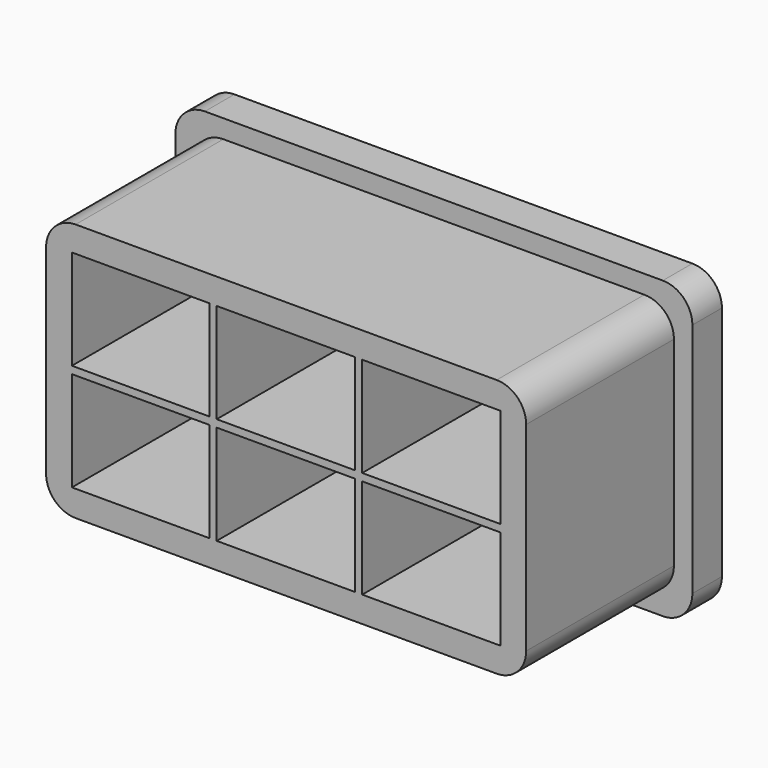
from build123d import *

# Parameters (mm, degrees)
F0_W     = 165.1
F0_H     = 88.9
F0_W_2   = 152.4
F0_H_2   = 76.2
F1_DEPTH = 76.2
F0_W_3   = 47.244
F0_H_3   = 34.29
F0_W_4   = 47.498
F2_DEPTH = 76.2
F3_R     = 10.16
F4_W     = 177.8
F4_H     = 101.6
F5_DEPTH = 12.7
F6_R     = 10.16


# Not quite as in the source:
# - a feature names something its author has since deleted; it is built from what else it names


with BuildPart() as f1:
    # F0 (on Front) → F1 (new body)
    with BuildSketch(Plane.XZ):
        Rectangle(F0_W, F0_H)
        Rectangle(F0_W_2, F0_H_2, mode=Mode.SUBTRACT)
    extrude(amount=F1_DEPTH)

    # F0 (on Front) → F2 (join)
    with BuildSketch(Plane.XZ):
        Rectangle(F0_W_2, F0_H_2)
        with Locations((-50.038, -18.415)):
            Rectangle(F0_W_3, F0_H_3, mode=Mode.SUBTRACT)
        with Locations((-0.127, -18.415)):
            Rectangle(F0_W_4, F0_H_3, mode=Mode.SUBTRACT)
        with Locations((49.911, -18.415)):
            Rectangle(F0_W_4, F0_H_3, mode=Mode.SUBTRACT)
        with Locations((-50.038, 18.415)):
            Rectangle(F0_W_3, F0_H_3, mode=Mode.SUBTRACT)
        with Locations((-0.127, 18.415)):
            Rectangle(F0_W_4, F0_H_3, mode=Mode.SUBTRACT)
        with Locations((49.911, 18.415)):
            Rectangle(F0_W_4, F0_H_3, mode=Mode.SUBTRACT)
    extrude(amount=F2_DEPTH)

    # F3
    f3_edges = [f1.edges().sort_by_distance(p)[0] for p in [
        (-82.55, -38.1, -44.45),
        (82.55, -38.1, -44.45),
        (-82.55, -38.1, 44.45),
        (82.55, -38.1, 44.45),
    ]]
    fillet(f3_edges, radius=F3_R)

    # F4 (on Front) → F5 (join)
    with BuildSketch(Plane.XZ):
        Rectangle(F4_W, F4_H)
    extrude(amount=F5_DEPTH)

    # F6
    f6_edges = [f1.edges().sort_by_distance(p)[0] for p in [
        (-88.9, -6.35, 50.8),
        (88.9, -6.35, 50.8),
        (-88.9, -6.35, -50.8),
        (88.9, -6.35, -50.8),
    ]]
    fillet(f6_edges, radius=F6_R)


solid = f1.part
